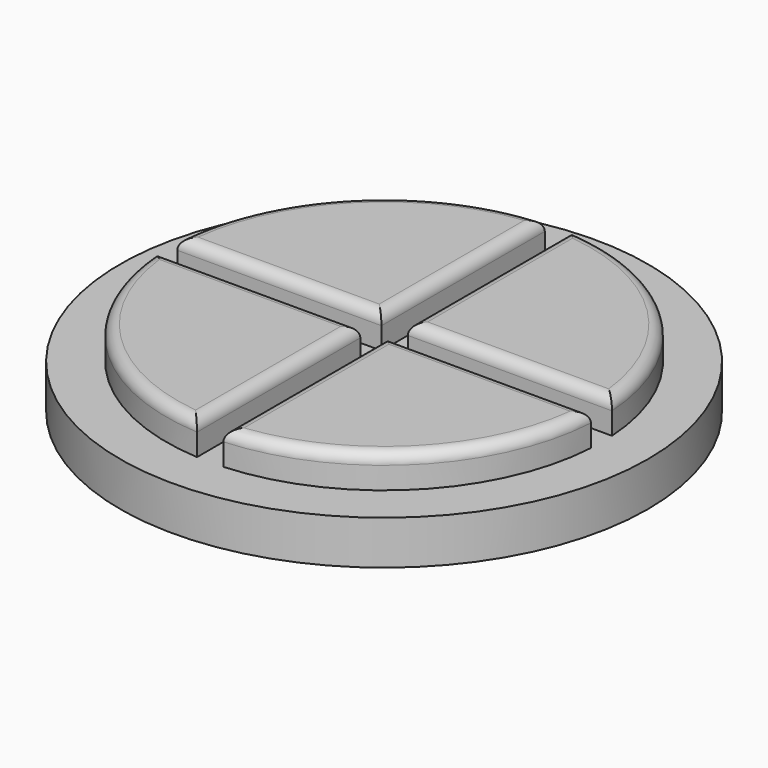
from build123d import *

# Parameters (mm, degrees)
F0_R     = 12
F1_DEPTH = 2
F3_DEPTH = 1.5
F4_R     = 0.5


with BuildPart() as f1:
    # F0 (on Top) → F1 (new body)
    with BuildSketch(Plane.XY):
        Circle(F0_R)
    extrude(amount=F1_DEPTH)

    # F2 (on face) → F3 (join)
    with BuildSketch(Plane.XY.offset(2)):
        with BuildLine():
            ThreePointArc((-9.8818014552, -0.6), (-7.0003571337, -7.0003571337), (-0.6, -9.8818014552))
            Line((-0.6, -9.8818014552), (-0.6, -0.6))
            Line((-0.6, -0.6), (-9.8818014552, -0.6))
        make_face()
        with BuildLine():
            Line((-0.6, 0.6), (-0.6, 9.8818014552))
            ThreePointArc((-0.6, 9.8818014552), (-7.0003571337, 7.0003571337), (-9.8818014552, 0.6))
            Line((-9.8818014552, 0.6), (-0.6, 0.6))
        make_face()
        with BuildLine():
            Line((0.6, 0.6), (9.8818014552, 0.6))
            ThreePointArc((9.8818014552, 0.6), (7.0003571337, 7.0003571337), (0.6, 9.8818014552))
            Line((0.6, 9.8818014552), (0.6, 0.6))
        make_face()
        with BuildLine():
            ThreePointArc((0.6, -9.8818014552), (7.0003571337, -7.0003571337), (9.8818014552, -0.6))
            Line((9.8818014552, -0.6), (0.6, -0.6))
            Line((0.6, -0.6), (0.6, -9.8818014552))
        make_face()
    extrude(amount=F3_DEPTH)

    # F4
    f4_edges = [f1.edges().sort_by_distance(p)[0] for p in [
        (-7.000357, -7.000357, 3.5),
        (-0.6, -5.240901, 3.5),
        (-5.240901, -0.6, 3.5),
        (-5.240901, 0.6, 3.5),
        (-0.6, 5.240901, 3.5),
        (5.240901, 0.6, 3.5),
        (0.6, 5.240901, 3.5),
        (5.240901, -0.6, 3.5),
        (0.6, -5.240901, 3.5),
        (7.000357, 7.000357, 3.5),
        (7.000357, -7.000357, 3.5),
        (-7.000357, 7.000357, 3.5),
    ]]
    fillet(f4_edges, radius=F4_R)


solid = f1.part
